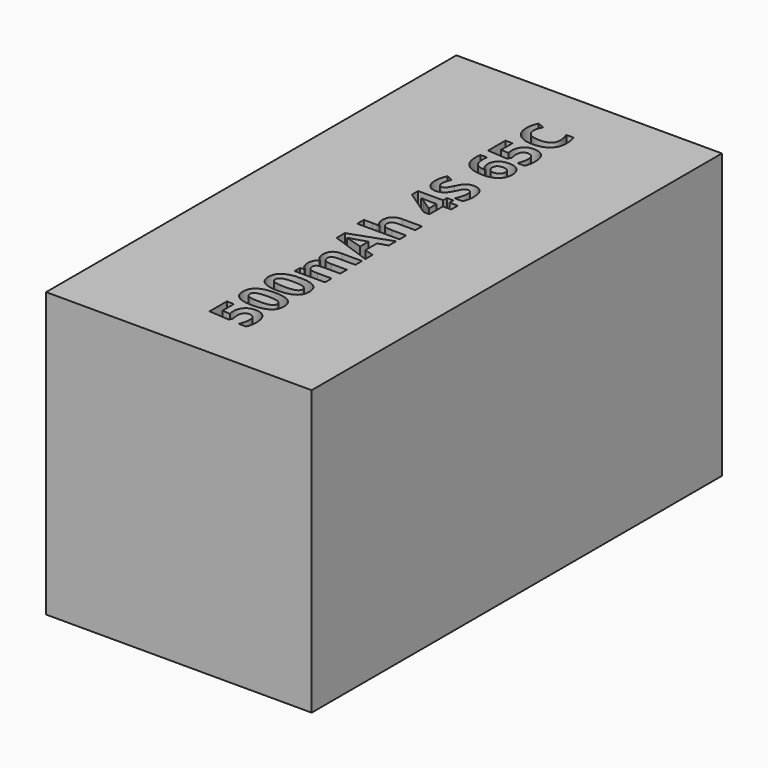
from build123d import *

# Parameters (mm, degrees)
F0_W         = 29
F0_H         = 56
F1_DEPTH     = 31
F2_TEXT_SIZE = 6.0801588309
F3_DEPTH     = 5


# Not quite as in the source:
# - Text() gives the source's letters only with a copy of the font that has no kerning and outlines rounded to 1/6400 em; it was checked with that copy


with BuildPart() as f1:
    # F0 (on Top) → F1 (new body)
    with BuildSketch(Plane.XY):
        Rectangle(F0_W, F0_H)
    extrude(amount=F1_DEPTH)

    # F2 (on face) → F3 (cut)
    with BuildSketch(Plane.XY.offset(31)):
        with Locations(Location((2.9457090914, -22.6103487164), (0, 0, 90))):
            Text('500mAh 4S 65C', F2_TEXT_SIZE, font='Open Sans', font_style=FontStyle.BOLD, text_align=(TextAlign.LEFT, TextAlign.BOTTOM))
    extrude(amount=-F3_DEPTH, mode=Mode.SUBTRACT)


solid = f1.part
